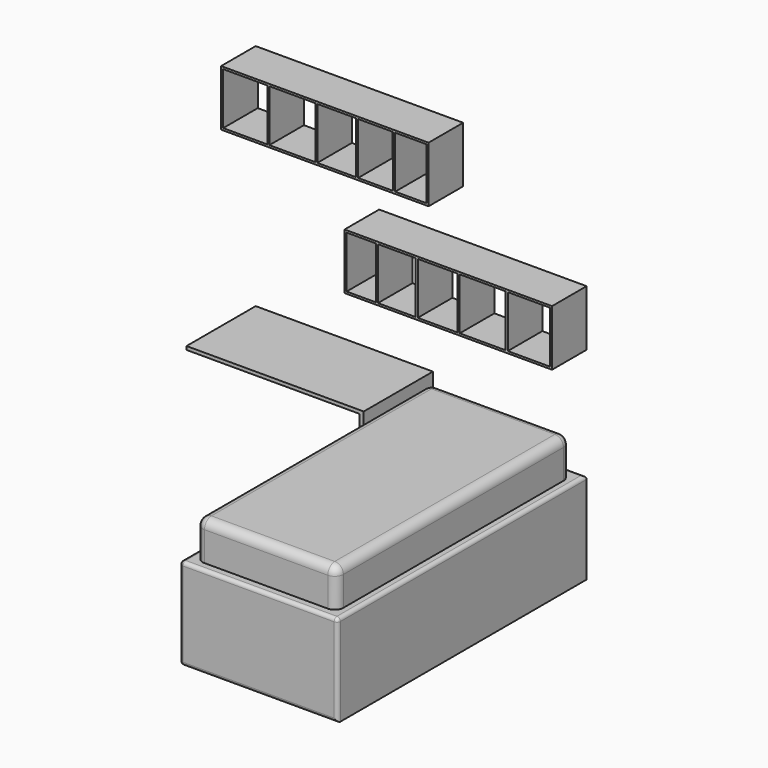
from build123d import *

# Parameters (mm, degrees)
F0_W      = 914
F0_H      = 750
F1_DEPTH  = 1800
F2_W      = 1000
F2_H      = 20
F3_DEPTH  = 500
F4_W      = 540
F4_H      = 210
F5_DEPTH  = 25
F6_W      = 914
F6_H      = 1800
F6_W_2    = 813.160777092
F6_H_2    = 1690.9182518721
F7_DEPTH  = 220
F8_W      = 1200
F8_H      = 324
F8_W_2    = 243.9199807754
F8_H_2    = 300
F8_W_3    = 265.7794940654
F8_W_4    = 230.8728685812
F8_W_5    = 218.2666818699
F8_W_6    = 169.1609747081
F9_DEPTH  = 250
F8_W_7    = 180.9111001602
F8_W_8    = 202.611290684
F8_W_9    = 223.7679018775
F8_W_10   = 265.6586144133
F8_W_11   = 255.051092865
F10_DEPTH = 25
F11_R     = 20
F12_R     = 50
F13_SIZE  = 10


# Not quite as in the source:
# - a feature names something its author has since deleted; it is built from what else it names


with BuildPart() as f1:
    # F0 (on Front) → F1 (new body)
    with BuildSketch(Plane.XZ):
        with Locations((1642, 375)):
            Rectangle(F0_W, F0_H)
    extrude(amount=F1_DEPTH)

    # F4 (on face) → F5 (join)
    with BuildSketch(Plane(origin=(1185, 0, 0), x_dir=(0, -1, 0), z_dir=(-1, 0, 0))):
        with Locations((1490, 145)):
            Rectangle(F4_W, F4_H)
        with Locations((330, 145)):
            Rectangle(F4_W, F4_H)
        with Locations((910, 145)):
            Rectangle(F4_W, F4_H)
        with Locations((1490, 395)):
            Rectangle(F4_W, F4_H)
        with Locations((330, 395)):
            Rectangle(F4_W, F4_H)
        with Locations((910, 395)):
            Rectangle(F4_W, F4_H)
    extrude(amount=F5_DEPTH)

    # F6 (on face) → F7 (cut)
    with BuildSketch(Plane.XY.offset(750)):
        with Locations((1642, -900)):
            Rectangle(F6_W, F6_H)
        with Locations((1643.2924866676, -901.5716090798)):
            Rectangle(F6_W_2, F6_H_2, mode=Mode.SUBTRACT)
    extrude(amount=-F7_DEPTH, mode=Mode.SUBTRACT)

    # F4 (on face) → F10 (join)
    with BuildSketch(Plane(origin=(1185, 0, 0), x_dir=(0, -1, 0), z_dir=(-1, 0, 0))):
        with Locations((1490, 145)):
            Rectangle(F4_W, F4_H)
        with Locations((330, 145)):
            Rectangle(F4_W, F4_H)
        with Locations((910, 145)):
            Rectangle(F4_W, F4_H)
        with Locations((1490, 395)):
            Rectangle(F4_W, F4_H)
        with Locations((330, 395)):
            Rectangle(F4_W, F4_H)
        with Locations((910, 395)):
            Rectangle(F4_W, F4_H)
    extrude(amount=F10_DEPTH)

    # F11
    f11_edges = [f1.edges().sort_by_distance(p)[0] for p in [
        (1642, -1800, 530),
        (1185, -900, 530),
        (1185, -1800, 265),
        (1185, 0, 265),
        (1642, 0, 530),
        (1642, -1800, 0),
        (1185, -900, 0),
        (2099, -900, 530),
        (2099, -1800, 265),
    ]]
    fillet(f11_edges, radius=F11_R)

    # F12
    f12_edges = [f1.edges().sort_by_distance(p)[0] for p in [
        (1236.712098, -901.571609, 750),
        (1643.292487, -1747.030735, 750),
        (1236.712098, -1747.030735, 640),
        (2049.872875, -1747.030735, 640),
        (2049.872875, -901.571609, 750),
        (1643.292487, -56.112483, 750),
        (2049.872875, -56.112483, 640),
        (1236.712098, -56.112483, 640),
    ]]
    fillet(f12_edges, radius=F12_R)

    # F13
    f13_edges = [f1.edges().sort_by_distance(p)[0] for p in [
        (1160, -330, 290),
        (1160, -600, 395),
        (1160, -330, 500),
        (1160, -60, 395),
        (1160, -910, 290),
        (1160, -1180, 395),
        (1160, -910, 500),
        (1160, -640, 395),
        (1160, -1490, 290),
        (1160, -1760, 395),
        (1160, -1490, 500),
        (1160, -1220, 395),
        (1160, -1490, 40),
        (1160, -1760, 145),
        (1160, -1490, 250),
        (1160, -1220, 145),
        (1160, -910, 40),
        (1160, -1180, 145),
        (1160, -910, 250),
        (1160, -640, 145),
        (1160, -330, 40),
        (1160, -600, 145),
        (1160, -330, 250),
        (1160, -60, 145),
    ]]
    chamfer(f13_edges, length=F13_SIZE)


with BuildPart() as f3:
    # F2 (on face) → F3 (new body)
    with BuildSketch(Plane(origin=(0, 0, 0), x_dir=(-1, 0, 0), z_dir=(0, 1, 0))):
        with Locations((-685, 760)):
            Rectangle(F2_W, F2_H)
        Polygon((-1185, 530), (-1185, 750), (-1185, 770), (-1210, 770), (-1210, 530), align=None)
    extrude(amount=-F3_DEPTH)


with BuildPart() as f9:
    # F8 (on face) → F9 (new body)
    with BuildSketch(Plane(origin=(0, 0, 0), x_dir=(-1, 0, 0), z_dir=(0, 1, 0))):
        with Locations((-1499, 1332)):
            Rectangle(F8_W, F8_H)
        with Locations((-1965.0400096123, 1332)):
            Rectangle(F8_W_2, F8_H_2, mode=Mode.SUBTRACT)
        with Locations((-1698.1902721919, 1332)):
            Rectangle(F8_W_3, F8_H_2, mode=Mode.SUBTRACT)
        with Locations((-1437.8640908686, 1332)):
            Rectangle(F8_W_4, F8_H_2, mode=Mode.SUBTRACT)
        with Locations((-1201.294315643, 1332)):
            Rectangle(F8_W_5, F8_H_2, mode=Mode.SUBTRACT)
        with Locations((-995.580487354, 1332)):
            Rectangle(F8_W_6, F8_H_2, mode=Mode.SUBTRACT)
    extrude(amount=-F9_DEPTH)


with BuildPart() as f9b:
    # F8 (on face) → F9, piece 2 (new body)
    with BuildSketch(Plane(origin=(0, 0, 0), x_dir=(-1, 0, 0), z_dir=(0, 1, 0))):
        with Locations((-785, 1932)):
            Rectangle(F8_W, F8_H)
        with Locations((-1282.5444499199, 1932)):
            Rectangle(F8_W_7, F8_H_2, mode=Mode.SUBTRACT)
        with Locations((-1078.7832544978, 1932)):
            Rectangle(F8_W_8, F8_H_2, mode=Mode.SUBTRACT)
        with Locations((-853.5936582171, 1932)):
            Rectangle(F8_W_9, F8_H_2, mode=Mode.SUBTRACT)
        with Locations((-596.8804000716, 1932)):
            Rectangle(F8_W_10, F8_H_2, mode=Mode.SUBTRACT)
        with Locations((-324.5255464325, 1932)):
            Rectangle(F8_W_11, F8_H_2, mode=Mode.SUBTRACT)
    extrude(amount=-F9_DEPTH)


solid = Compound([f1.part, f3.part, f9.part, f9b.part])
